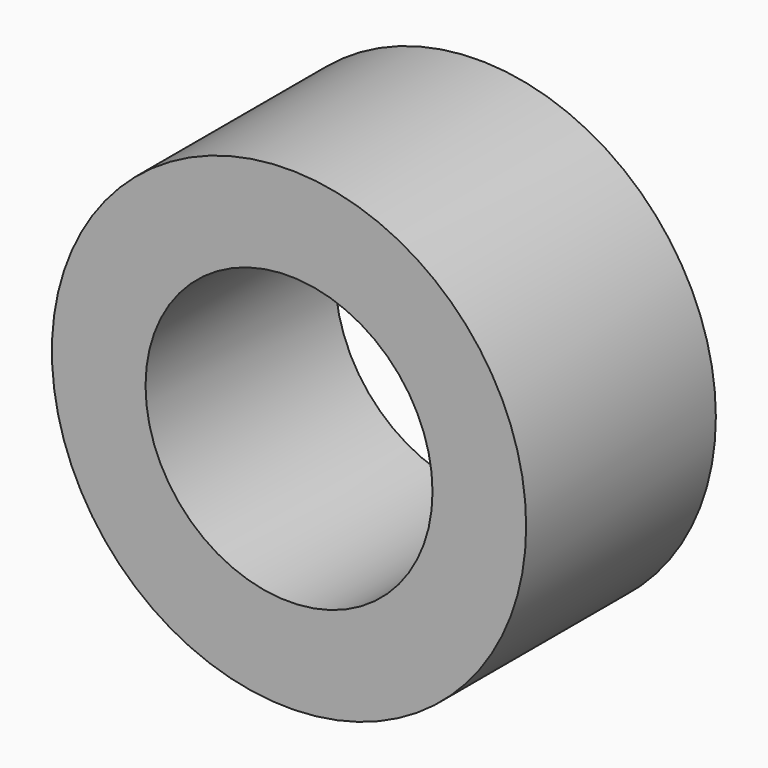
from build123d import *

# Parameters (mm, degrees)
F0_R     = 25
F0_R_2   = 15.1279362517
F1_DEPTH = 25


with BuildPart() as f1:
    # F0 (on Front) → F1 (new body)
    with BuildSketch(Plane.XZ):
        Circle(F0_R)
        Circle(F0_R_2, mode=Mode.SUBTRACT)
    extrude(amount=F1_DEPTH)


solid = f1.part
